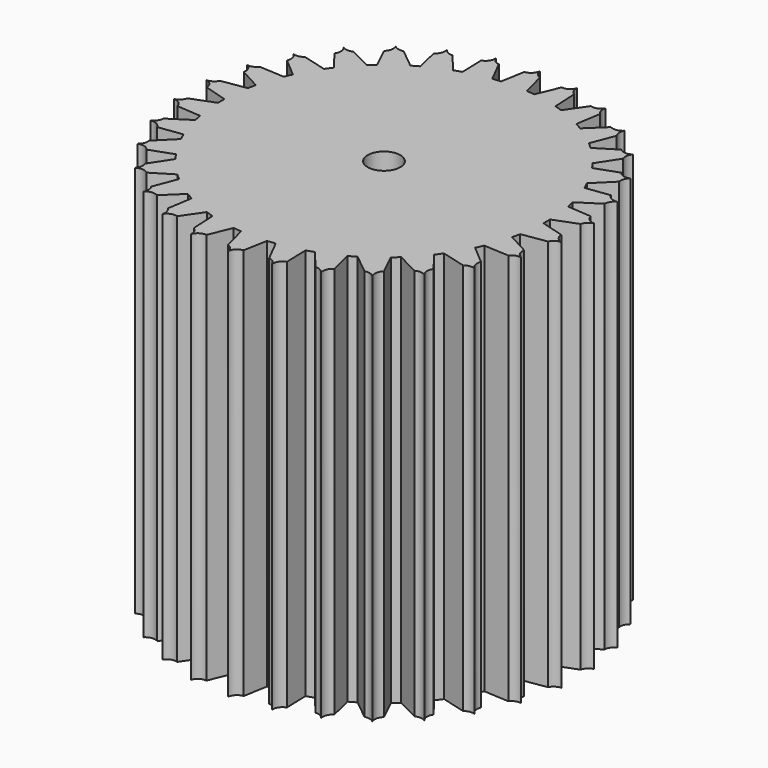
from build123d import *

# Parameters (mm, degrees)
F0_R            = 7.62
F1_DEPTH        = 7.62
F2_R            = 0.635
F3_DEPTH        = 15.24
F5_DEPTH        = 15.24
F5_COPIES_COUNT = 30


# Not quite as in the source:
# - a pattern or mirror of a feature is missing from the dataset's text; its kind, count and spacing are read off the source's solid


with BuildPart() as f1:
    # F0 (on Top) → F1 (new body, symmetric)
    with BuildSketch(Plane.XY):
        Circle(F0_R)
    extrude(amount=F1_DEPTH, both=True)

    # F2 (on face) → F3 (cut, through all)
    with BuildSketch(Plane.XY.offset(7.62)):
        Circle(F2_R)
    extrude(amount=-F3_DEPTH, mode=Mode.SUBTRACT)

    # F4 (on face) → F5 (cut, through all)
    with BuildSketch(Plane.XY.offset(7.62)):
        with BuildLine():
            ThreePointArc((1.1774650041, 7.1433782284), (1.4434722472, 7.2178126365), (1.5892749077, 7.4524227784))
            ThreePointArc((1.5892749077, 7.4524227784), (0.7990426862, 7.5779898908), (0, 7.62))
            ThreePointArc((0, 7.62), (0.0679999401, 7.3924435649), (0.2571516718, 7.248820637))
            Line((0.2571516718, 7.248820637), (0.508, 6.3051195791))
            ThreePointArc((0.508, 6.3051195791), (0.6637440585, 6.290631187), (0.8190822636, 6.2722963221))
            Line((0.8190822636, 6.2722963221), (1.1774650041, 7.1433782284))
        make_face()
    f5 = extrude(amount=-F5_DEPTH, mode=Mode.SUBTRACT)

    # F5_copies: F5 ×30 about axis
    f5_copies_axis = Axis((0, 0, 0), (0, 0, 1))
    for i in range(1, F5_COPIES_COUNT):
        add(f5.rotate(f5_copies_axis, i * 360 / F5_COPIES_COUNT), mode=Mode.SUBTRACT)


solid = f1.part
